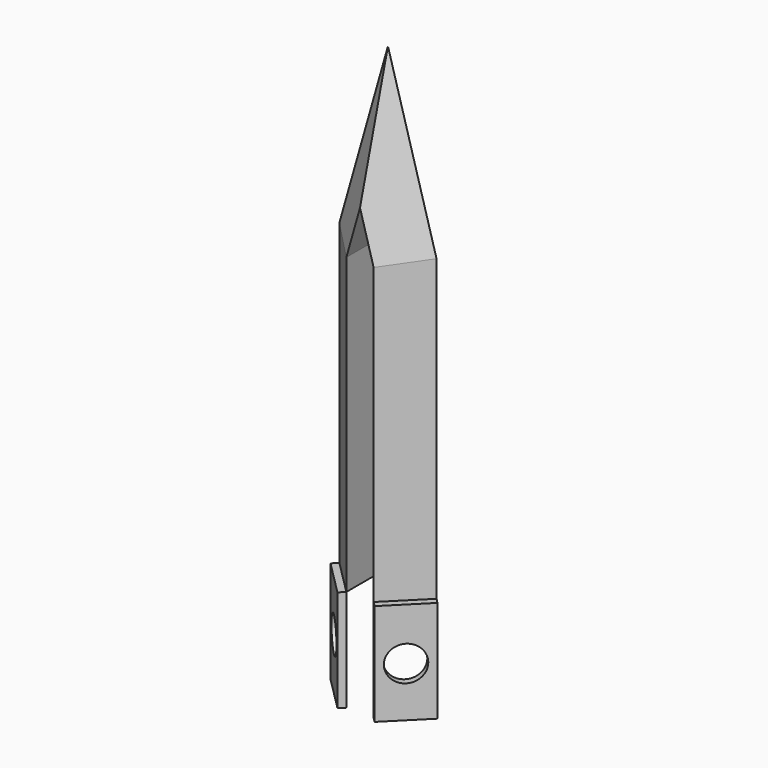
from build123d import *

# Parameters (mm, degrees)
F1_DEPTH  = 2.54
F2_SIZE   = 2.53999
F7_DEPTH  = 22.86
F8_R      = 1.27
F9_DEPTH  = 0.508
F6_R      = 1.27
F10_DEPTH = 0.508


# Not quite as in the source:
# - a fillet or chamfer is up to 0.001 mm smaller than in the source, because OpenCascade refuses the exact size
# - ends of sketch curves that miss each other by under 0.0002 mm in the source are joined


with BuildPart() as f1:
    # F0 (on Front) → F1 (new body)
    with BuildSketch(Plane.XZ):
        Polygon((-2.687785076, 12.45414), (-6.2184794806, 0), (-6.2184794806, -21.7626541853), (-2.687785076, -21.7626541853), align=None)
    extrude(amount=F1_DEPTH)

    # F2 (size 2.54 in the source; OpenCascade refuses exactly that, so slightly less here)
    f2_edges = [f1.edges().sort_by_distance(p)[0] for p in [
        (-6.218479, -2.54, -10.881327),
        (-4.453132, -2.54, 6.22707),
    ]]
    chamfer(f2_edges, length=F2_SIZE)

    # F3: F1 across face


with BuildPart() as f1_1:
    add(f1.part)
    add(f1.part.mirror(Plane(origin=(-4.3222158923, 0, -7.5368954457), x_dir=(1, 0, 0), z_dir=(0, 1, 0))))

    # F4: F1 across face


with BuildPart() as f1_2:
    add(f1_1.part)
    add(f1_1.part.mirror(Plane(origin=(-2.687785076, 0, -6.8601697168), x_dir=(0, 1, 0), z_dir=(1, 0, 0))))

    # F5 (on face) → F7 (cut)
    with BuildSketch(Plane.XZ.offset(2.54)):
        Polygon((-1.6970906714, -0.3530822644), (-2.687785076, 3.1414843557), (-3.6784794806, -0.3530822644), (-3.6784794806, -21.7626541853), (-1.6970806714, -21.7626541853), align=None)
    extrude(amount=-F7_DEPTH, mode=Mode.SUBTRACT)


with BuildPart() as f9:
    # F8 (on face) → F9 (new body)
    with BuildSketch(Plane(origin=(-3.1092397403, -3.1092397403, 0), x_dir=(0.7071067812, -0.7071067812, 0), z_dir=(-0.7071067812, -0.7071067812, 0))):
        Polygon((-0.805033632, -21.7626541853), (-4.3971219383, -21.7626541853), (-4.3971290094, -29.1721168905), (-0.805026561, -29.1721168905), align=None)
        with Locations((-2.6010777852, -25.3909938037)):
            Circle(F8_R, mode=Mode.SUBTRACT)
    extrude(amount=F9_DEPTH)


with BuildPart() as f10:
    # F6 (on face) → F10 (new body)
    with BuildSketch(Plane(origin=(0.4214546643, -0.4214546643, 0), x_dir=(0.7071067812, 0.7071067812, 0), z_dir=(0.7071067812, -0.7071067812, 0))):
        Polygon((0.5960198311, -21.7626541853), (-2.9960684752, -21.7626541853), (-2.9960755462, -29.1721135853), (0.5960269022, -29.1721135853), align=None)
        with Locations((-1.200024322, -25.5403872579)):
            Circle(F6_R, mode=Mode.SUBTRACT)
    extrude(amount=F10_DEPTH)


solid = Compound([f1_2.part, f9.part, f10.part])
